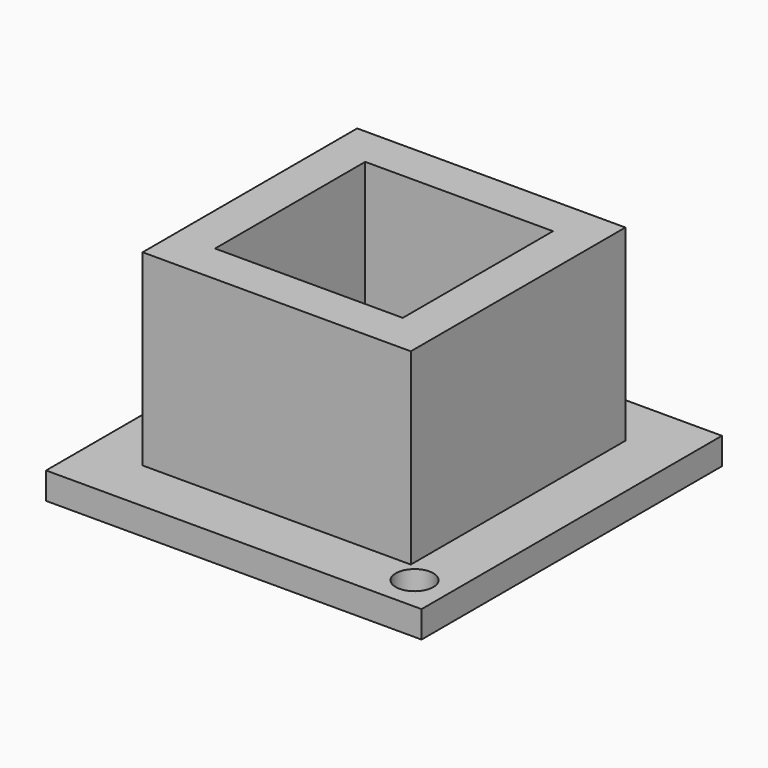
from build123d import *

# Parameters (mm, degrees)
F0_W     = 70
F0_H     = 70
F0_R     = 3.5
F0_R_2   = 12.7
F1_DEPTH = 5
F2_W     = 50
F2_H     = 50
F2_W_2   = 35
F2_H_2   = 35
F3_DEPTH = 35
F4_R     = 13.4
F4_R_2   = 12.7
F5_DEPTH = 2.5


# Not quite as in the source:
# - a feature names something its author has since deleted; it is built from what else it names


with BuildPart() as f1:
    # F0 (on Top) → F1 (new body)
    with BuildSketch(Plane.XY):
        Rectangle(F0_W, F0_H)
        with Locations((28.5, -28.5)):
            Circle(F0_R, mode=Mode.SUBTRACT)
        with Locations((-28.5, 28.5)):
            Circle(F0_R, mode=Mode.SUBTRACT)
        Circle(F0_R_2, mode=Mode.SUBTRACT)
    extrude(amount=F1_DEPTH)

    # F2 (on face) → F3 (join)
    with BuildSketch(Plane.XY.offset(5)):
        Rectangle(F2_W, F2_H)
        Rectangle(F2_W_2, F2_H_2, mode=Mode.SUBTRACT)
    extrude(amount=F3_DEPTH)

    # F4 (on face) → F5 (cut)
    with BuildSketch(Plane(origin=(0, 0, 0), x_dir=(1, 0, 0), z_dir=(0, 0, -1))):
        Circle(F4_R)
        Circle(F4_R_2, mode=Mode.SUBTRACT)
    extrude(amount=-F5_DEPTH, mode=Mode.SUBTRACT)


solid = f1.part
